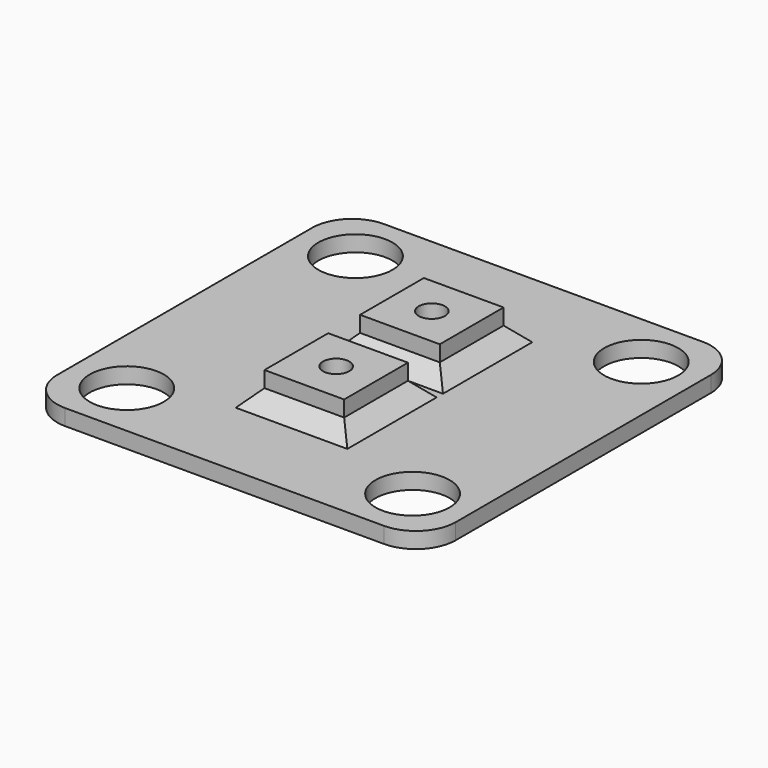
from build123d import *

# Parameters (mm, degrees)
F0_W     = 10
F0_H     = 10
F0_R     = 1.65
F1_DEPTH = 6
F0_R_2   = 4.65
F2_DEPTH = 2
F3_SIZE  = 2


with BuildPart() as f1:
    # F0 (on Top) → F1 (new body)
    with BuildSketch(Plane.XY):
        with Locations((0, 7.5)):
            Rectangle(F0_W, F0_H)
        with Locations((0, 7.5)):
            Circle(F0_R, mode=Mode.SUBTRACT)
    extrude(amount=F1_DEPTH)



with BuildPart() as f1b:
    # F0 (on Top) → F1, piece 2 (new body)
    with BuildSketch(Plane.XY):
        with Locations((0, -7.5)):
            Rectangle(F0_W, F0_H)
        with Locations((0, -7.5)):
            Circle(F0_R, mode=Mode.SUBTRACT)
    extrude(amount=F1_DEPTH)


with BuildPart() as f1_1:
    add(f1.part)

    add(f1b.part)  # F2 merges F1b
    # F0 (on Top) → F2 (join)
    with BuildSketch(Plane.XY):
        with BuildLine():
            Line((20, 25), (-20, 25))
            ThreePointArc((-20, 25), (-23.5355339059, 23.5355339059), (-25, 20))
            Line((-25, 20), (-25, -20))
            ThreePointArc((-25, -20), (-23.5355339059, -23.5355339059), (-20, -25))
            Line((-20, -25), (20, -25))
            ThreePointArc((20, -25), (23.5355339059, -23.5355339059), (25, -20))
            Line((25, -20), (25, 20))
            ThreePointArc((25, 20), (23.5355339059, 23.5355339059), (20, 25))
        make_face()
        with Locations((-17.9289321881, -17.9289321881)):
            Circle(F0_R_2, mode=Mode.SUBTRACT)
        with Locations((17.9289321881, -17.9289321881)):
            Circle(F0_R_2, mode=Mode.SUBTRACT)
        with Locations((0, -7.5)):
            Rectangle(F0_W, F0_H, mode=Mode.SUBTRACT)
        with Locations((-17.9289321881, 17.9289321881)):
            Circle(F0_R_2, mode=Mode.SUBTRACT)
        with Locations((0, 7.5)):
            Rectangle(F0_W, F0_H, mode=Mode.SUBTRACT)
        with Locations((17.9289321881, 17.9289321881)):
            Circle(F0_R_2, mode=Mode.SUBTRACT)
    extrude(amount=F2_DEPTH)

    # F3
    f3_edges = [f1_1.edges().sort_by_distance(p)[0] for p in [
        (0, -12.5, 2),
        (5, -7.5, 2),
        (5, 7.5, 2),
        (0, 2.5, 2),
        (0, -2.5, 2),
        (0, 12.5, 2),
        (-5, 7.5, 2),
        (-5, -7.5, 2),
    ]]
    chamfer(f3_edges, length=F3_SIZE)


solid = f1_1.part
